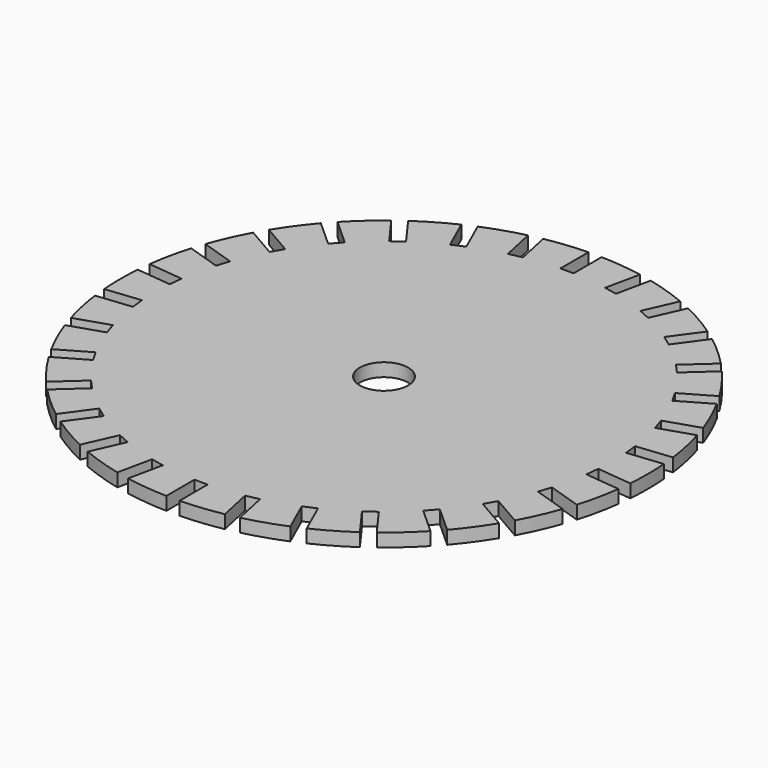
from build123d import *

# Parameters (mm, degrees)
F0_R            = 60
F0_R_2          = 5.5
F1_DEPTH        = 3
F3_DEPTH        = 25
F3_COPIES_COUNT = 30


# Not quite as in the source:
# - a pattern or mirror of a feature is missing from the dataset's text; its kind, count and spacing are read off the source's solid


with BuildPart() as f1:
    # F0 (on Top) → F1 (new body)
    with BuildSketch(Plane.XY):
        Circle(F0_R)
        Circle(F0_R_2, mode=Mode.SUBTRACT)
    extrude(amount=F1_DEPTH)

    # F2 (on Top) → F3 (cut)
    with BuildSketch(Plane.XY):
        Polygon((-1.5, -60), (0, -60), (1.5, -60), (1.5, -52), (-1.5, -52), align=None)
    f3 = extrude(amount=F3_DEPTH, mode=Mode.SUBTRACT)

    # F3_copies: F3 ×30 about axis
    f3_copies_axis = Axis((0, 0, 0), (0, 0, 1))
    for i in range(1, F3_COPIES_COUNT):
        add(f3.rotate(f3_copies_axis, i * 360 / F3_COPIES_COUNT), mode=Mode.SUBTRACT)


solid = f1.part
